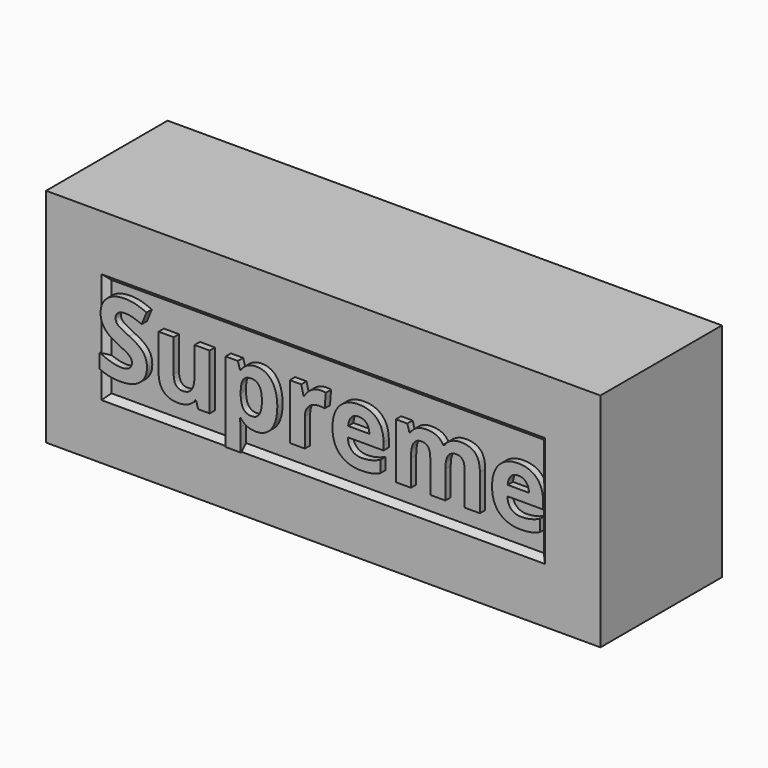
from build123d import *

# Parameters (mm, degrees)
F0_W         = 127
F0_H         = 50.8
F1_DEPTH     = 34.798
F2_W         = 104.14
F2_H         = 27.94
F3_DEPTH     = 1.27
F4_TEXT_SIZE = 23.2447250026
F5_DEPTH     = 1.524
F6_T4_DEPTH  = 117.2041495789
F6_T9_DEPTH  = 117.2041495789
F7_T4_DEPTH  = 35.9241495789
F7_T9_DEPTH  = 35.9241495789


# Not quite as in the source:
# - a fillet or chamfer that OpenCascade refuses, or shapes differently, is made with other operations: its cross-section is extruded or revolved along the edge and cut away or added
# - a feature names something its author has since deleted; it is built from what else it names
# - Text() gives the source's letters only with a copy of the font that has no kerning and outlines rounded to 1/6400 em; it was checked with that copy


with BuildPart() as f1:
    # F0 (on Front) → F1 (new body)
    with BuildSketch(Plane.XZ):
        with Locations((-63.5, -25.4)):
            Rectangle(F0_W, F0_H)
    extrude(amount=F1_DEPTH)

    # F2 (on face) → F3 (cut)
    with BuildSketch(Plane.XZ.offset(34.798)):
        with Locations((-63.5, -25.4)):
            Rectangle(F2_W, F2_H)
    extrude(amount=-F3_DEPTH, mode=Mode.SUBTRACT)

    # F4 (on face) → F5 (join)
    with BuildSketch(Plane.XZ.offset(33.528)):
        with Locations((-115.57, -32.5588539132)):
            Text('Supreme', F4_TEXT_SIZE, font='Open Sans', font_style=FontStyle.BOLD, text_align=(TextAlign.LEFT, TextAlign.BOTTOM))
    extrude(amount=F5_DEPTH)

    # F6: chamfer of 2.54 on 2 edges, made by hand


with BuildPart() as f6_tool2:
    # F6_s3 → F6_t4 (new body)
    with BuildSketch(Plane.YZ.offset(-4.8979252106)):
        Polygon((-36.068, -11.43), (-33.528, -13.97), (-33.528, -11.43), align=None)
    extrude(amount=-F6_T4_DEPTH)

    split(bisect_by=Plane.XZ.offset(34.798), keep=Keep.BOTTOM)


with BuildPart() as f1_1:
    add(f1.part)

    # F6_t1: union F6_tool2
    add(f6_tool2.part)


with BuildPart() as f6_tool7:
    # F6_s8 → F6_t9 (new body)
    with BuildSketch(Plane.YZ.offset(-122.1020747894)):
        Polygon((-36.068, -39.37), (-33.528, -36.83), (-33.528, -39.37), align=None)
    extrude(amount=F6_T9_DEPTH)

    split(bisect_by=Plane.XZ.offset(34.798), keep=Keep.BOTTOM)


with BuildPart() as f1_2:
    add(f1_1.part)

    # F6_t6: union F6_tool7
    add(f6_tool7.part)

    # F7: chamfer of 2.54 on 2 edges, made by hand


with BuildPart() as f7_tool2:
    # F7_s3 → F7_t4 (new body)
    with BuildSketch(Plane.XY.offset(-43.3620747894)):
        Polygon((-11.43, -36.068), (-13.97, -33.528), (-11.43, -33.528), align=None)
    extrude(amount=F7_T4_DEPTH)

    split(bisect_by=Plane.XZ.offset(34.798), keep=Keep.BOTTOM)


with BuildPart() as f1_3:
    add(f1_2.part)

    # F7_t1: union F7_tool2
    add(f7_tool2.part)


with BuildPart() as f7_tool7:
    # F7_s8 → F7_t9 (new body)
    with BuildSketch(Plane.XY.offset(-7.4379252106)):
        Polygon((-115.57, -36.068), (-113.03, -33.528), (-115.57, -33.528), align=None)
    extrude(amount=-F7_T9_DEPTH)

    split(bisect_by=Plane.XZ.offset(34.798), keep=Keep.BOTTOM)


with BuildPart() as f1_4:
    add(f1_3.part)

    # F7_t6: union F7_tool7
    add(f7_tool7.part)


solid = f1_4.part
